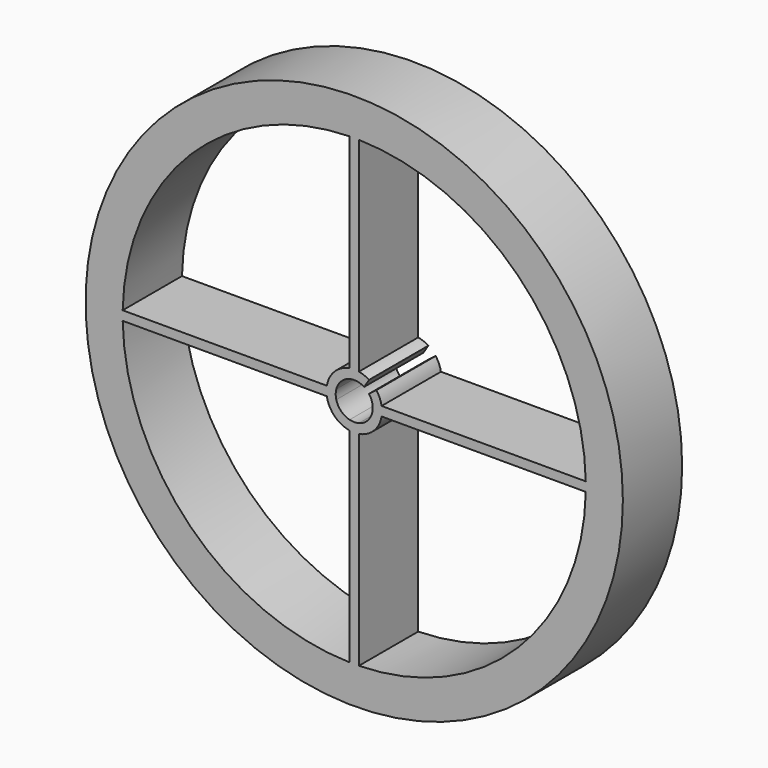
from build123d import *

# Parameters (mm, degrees)
F0_R     = 29
F1_DEPTH = 8


with BuildPart() as f1:
    # F0 (on Front) → F1 (new body)
    with BuildSketch(Plane.XZ):
        Circle(F0_R)
        with BuildLine():
            ThreePointArc((0.5, 24.9949994999), (17.6776695297, 17.6776695297), (24.9949994999, 0.5))
            ThreePointArc((24.9949994999, 0.5), (24.9987498437, 0.2500125022), (25, 0))
            ThreePointArc((25, 0), (24.9987498437, -0.2500125022), (24.9949994999, -0.5))
            ThreePointArc((24.9949994999, -0.5), (17.6776695297, -17.6776695297), (0.5, -24.9949994999))
            ThreePointArc((0.5, -24.9949994999), (0, -25), (-0.5, -24.9949994999))
            ThreePointArc((-0.5, -24.9949994999), (-17.6776695297, -17.6776695297), (-24.9949994999, -0.5))
            ThreePointArc((-24.9949994999, -0.5), (-25, 0), (-24.9949994999, 0.5))
            ThreePointArc((-24.9949994999, 0.5), (-17.6776695297, 17.6776695297), (-0.5, 24.9949994999))
            ThreePointArc((-0.5, 24.9949994999), (0, 25), (0.5, 24.9949994999))
        make_face(mode=Mode.SUBTRACT)
        with BuildLine():
            ThreePointArc((1.9364916731, 0.5), (1.9840593925, 0.252008585), (2, 0))
            ThreePointArc((2, 0), (1.9840593925, -0.252008585), (1.9364916731, -0.5))
            Line((1.9364916731, -0.5), (2.9580398915, -0.5))
            ThreePointArc((2.9580398915, -0.5), (2.9894915684, -0.2508787808), (3, 0))
            ThreePointArc((3, 0), (2.9894915684, 0.2508787808), (2.9580398915, 0.5))
            Line((2.9580398915, 0.5), (1.9364916731, 0.5))
        make_face()
        with BuildLine():
            ThreePointArc((1.5931753199, 1.2090460702), (1.8000899569, 0.8715940265), (1.9364916731, 0.5))
            Line((1.9364916731, 0.5), (2.9580398915, 0.5))
            ThreePointArc((2.9580398915, 0.5), (2.7533824356, 1.1911696619), (2.3897629799, 1.8135691053))
            Line((2.3897629799, 1.8135691053), (1.5931753199, 1.2090460702))
        make_face()
        with BuildLine():
            Line((2.9580398915, -0.5), (1.9364916731, -0.5))
            ThreePointArc((1.9364916731, -0.5), (1.4142135624, -1.4142135624), (0.5, -1.9364916731))
            Line((0.5, -1.9364916731), (0.5, -2.9580398915))
            ThreePointArc((0.5, -2.9580398915), (2.1213203436, -2.1213203436), (2.9580398915, -0.5))
        make_face()
        with BuildLine():
            Line((24.9949994999, 0.5), (2.9580398915, 0.5))
            ThreePointArc((2.9580398915, 0.5), (2.9894915684, 0.2508787808), (3, 0))
            ThreePointArc((3, 0), (2.9894915684, -0.2508787808), (2.9580398915, -0.5))
            Line((2.9580398915, -0.5), (24.9949994999, -0.5))
            ThreePointArc((24.9949994999, -0.5), (24.9987498437, -0.2500125022), (25, 0))
            ThreePointArc((25, 0), (24.9987498437, 0.2500125022), (24.9949994999, 0.5))
        make_face()
        with BuildLine():
            Line((0.5, -2.9580398915), (0.5, -1.9364916731))
            ThreePointArc((0.5, -1.9364916731), (0, -2), (-0.5, -1.9364916731))
            Line((-0.5, -1.9364916731), (-0.5, -2.9580398915))
            ThreePointArc((-0.5, -2.9580398915), (0, -3), (0.5, -2.9580398915))
        make_face()
        with BuildLine():
            ThreePointArc((0.5, 1.9364916731), (0.7937447605, 1.8357476012), (1.068353257, 1.6907457876))
            Line((1.068353257, 1.6907457876), (1.6025298855, 2.5361186814))
            ThreePointArc((1.6025298855, 2.5361186814), (1.0722230909, 2.8018453996), (0.5, 2.9580398915))
            Line((0.5, 2.9580398915), (0.5, 1.9364916731))
        make_face()
        with BuildLine():
            Line((-0.5, -2.9580398915), (-0.5, -1.9364916731))
            ThreePointArc((-0.5, -1.9364916731), (-1.4142135624, -1.4142135624), (-1.9364916731, -0.5))
            Line((-1.9364916731, -0.5), (-2.9580398915, -0.5))
            ThreePointArc((-2.9580398915, -0.5), (-2.1213203436, -2.1213203436), (-0.5, -2.9580398915))
        make_face()
        with BuildLine():
            Line((0.5, -24.9949994999), (0.5, -2.9580398915))
            ThreePointArc((0.5, -2.9580398915), (0, -3), (-0.5, -2.9580398915))
            Line((-0.5, -2.9580398915), (-0.5, -24.9949994999))
            ThreePointArc((-0.5, -24.9949994999), (0, -25), (0.5, -24.9949994999))
        make_face()
        with BuildLine():
            ThreePointArc((-0.5, 1.9364916731), (0, 2), (0.5, 1.9364916731))
            Line((0.5, 1.9364916731), (0.5, 2.9580398915))
            ThreePointArc((0.5, 2.9580398915), (0, 3), (-0.5, 2.9580398915))
            Line((-0.5, 2.9580398915), (-0.5, 1.9364916731))
        make_face()
        with BuildLine():
            Line((0.5, 2.9580398915), (0.5, 24.9949994999))
            ThreePointArc((0.5, 24.9949994999), (0, 25), (-0.5, 24.9949994999))
            Line((-0.5, 24.9949994999), (-0.5, 2.9580398915))
            ThreePointArc((-0.5, 2.9580398915), (0, 3), (0.5, 2.9580398915))
        make_face()
        with BuildLine():
            Line((-2.9580398915, -0.5), (-1.9364916731, -0.5))
            ThreePointArc((-1.9364916731, -0.5), (-2, 0), (-1.9364916731, 0.5))
            Line((-1.9364916731, 0.5), (-2.9580398915, 0.5))
            ThreePointArc((-2.9580398915, 0.5), (-3, 0), (-2.9580398915, -0.5))
        make_face()
        with BuildLine():
            ThreePointArc((-1.9364916731, 0.5), (-1.4142135624, 1.4142135624), (-0.5, 1.9364916731))
            Line((-0.5, 1.9364916731), (-0.5, 2.9580398915))
            ThreePointArc((-0.5, 2.9580398915), (-2.1213203436, 2.1213203436), (-2.9580398915, 0.5))
            Line((-2.9580398915, 0.5), (-1.9364916731, 0.5))
        make_face()
        with BuildLine():
            Line((-24.9949994999, -0.5), (-2.9580398915, -0.5))
            ThreePointArc((-2.9580398915, -0.5), (-3, 0), (-2.9580398915, 0.5))
            Line((-2.9580398915, 0.5), (-24.9949994999, 0.5))
            ThreePointArc((-24.9949994999, 0.5), (-25, 0), (-24.9949994999, -0.5))
        make_face()
    extrude(amount=F1_DEPTH)


solid = f1.part
